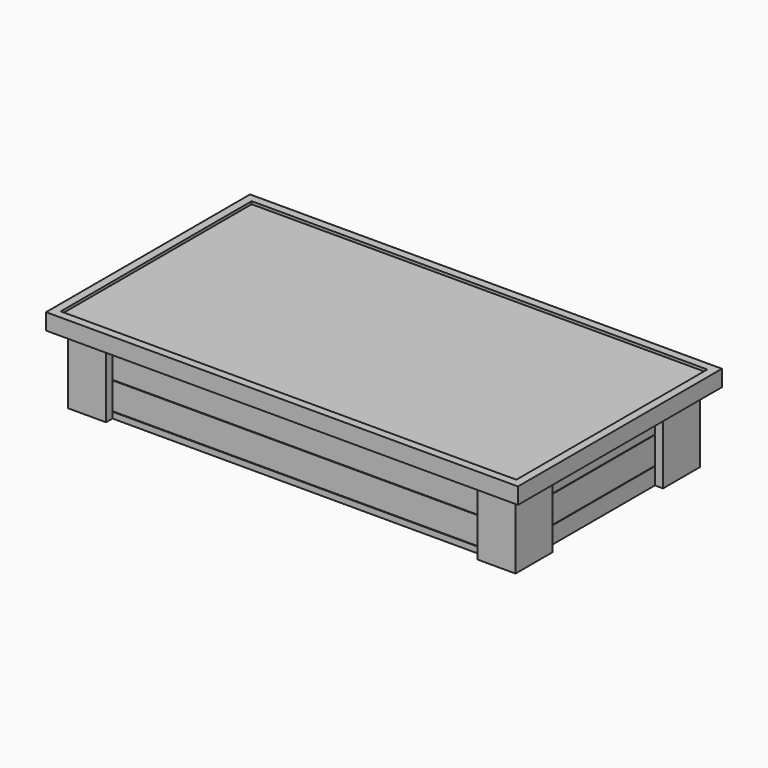
from build123d import *

# Parameters (mm, degrees)
F0_W      = 1066.8
F0_H      = 558.8
F1_DEPTH  = 6.35
F3_W      = 1104.9
F3_H      = 596.9
F3_W_2    = 1066.8
F3_H_2    = 558.8
F4_DEPTH  = 38.1
F5_W      = 1066.8
F5_H      = 558.8
F6_DEPTH  = 19.05
F7_W      = 872.49
F7_H      = 19.05
F8_DEPTH  = 88.9
F9_W      = 38.1
F9_H      = 63.5
F10_DEPTH = 457.2
F11_W     = 19.05
F11_H     = 88.9
F12_DEPTH = 419.1
F14_DEPTH = 192.786
F15_W     = 323.85
F15_H     = 1.143
F15_W_2   = 329.2250932205
F16_DEPTH = 1219.2
F17_W     = 869.95
F17_H     = 1.143
F18_DEPTH = 25.4
F20_W     = 872.49
F20_H     = 19.05
F21_DEPTH = 128.143
F22_W     = 869.95
F22_H     = 1.143
F23_DEPTH = 25.4
F24_W     = 38.1
F24_H     = 88.9
F25_DEPTH = 226.314
F26_W     = 558.8
F26_H     = 381
F27_DEPTH = 1397


# Not quite as in the source:
# - a feature of the source that left no trace in its solid (it failed there, or was rolled back) is left out


with BuildPart() as f1:
    # F0 (on Top) → F1 (new body)
    with BuildSketch(Plane.XY):
        with Locations((32.4463618145, 18.8094943296)):
            Rectangle(F0_W, F0_H)
    extrude(amount=F1_DEPTH)


with BuildPart() as f4:
    # F3 (on offset) → F4 (new body)
    with BuildSketch(Plane.XY.offset(12.7)):
        with Locations((32.4463618145, 18.8094943296)):
            Rectangle(F3_W, F3_H)
        with Locations((32.4463618145, 18.8094943296)):
            Rectangle(F3_W_2, F3_H_2, mode=Mode.SUBTRACT)
    extrude(amount=-F4_DEPTH)


with BuildPart() as f6:
    # F5 (on face) → F6 (new body)
    with BuildSketch(Plane(origin=(0, 0, 0), x_dir=(1, 0, 0), z_dir=(0, 0, -1))):
        with Locations((32.4463618145, -18.8094943296)):
            Rectangle(F5_W, F5_H)
        Polygon((-462.8536381855, -233.1854943296), (-462.8536381855, 195.5665056704), (-9.4854419759, -18.8094943296), align=None, mode=Mode.SUBTRACT)
        Polygon((32.4463618145, -38.6370262221), (500.8223618145, -260.1094943296), (-435.9296381855, -260.1094943296), align=None, mode=Mode.SUBTRACT)
        Polygon((-435.9296381855, 222.4905056704), (500.8223618145, 222.4905056704), (32.4463618145, 1.0180375628), align=None, mode=Mode.SUBTRACT)
        Polygon((74.378165605, -18.8094943296), (527.7463618145, 195.5665056704), (527.7463618145, -233.1854943296), align=None, mode=Mode.SUBTRACT)
    extrude(amount=F6_DEPTH)

    # F7 (on face) → F8 (join)
    with BuildSketch(Plane(origin=(0, 0, -19.05), x_dir=(1, 0, 0), z_dir=(0, 0, -1))):
        with Locations((32.4463618145, 222.4905056704)):
            Rectangle(F7_W, F7_H)
    extrude(amount=F8_DEPTH)

    # F9 (on face) → F10 (join)
    with BuildSketch(Plane(origin=(0, -212.9655056704, 0), x_dir=(-1, 0, 0), z_dir=(0, 1, 0))):
        with Locations((384.7486381855, -50.8)):
            Rectangle(F9_W, F9_H)
        with Locations((-449.6413618145, -50.8)):
            Rectangle(F9_W, F9_H)
    extrude(amount=F10_DEPTH)

    # F11 (on face) → F12 (join)
    with BuildSketch(Plane(origin=(0, 0, -19.05), x_dir=(1, 0, 0), z_dir=(0, 0, -1))):
        Polygon((-402.5286381855, 251.0655056704), (-491.4286381855, 251.0655056704), (-491.4286381855, 232.0155056704), (-472.3786381855, 232.0155056704), (-402.5286381855, 232.0155056704), align=None)
        with Locations((-481.9036381855, 187.5655056704)):
            Rectangle(F11_W, F11_H)
        Polygon((-491.4286381855, -269.6344943296), (-491.4286381855, -288.6844943296), (-402.5286381855, -288.6844943296), (-402.5286381855, -269.6344943296), (-472.3786381855, -269.6344943296), align=None)
        with Locations((-481.9036381855, -225.1844943296)):
            Rectangle(F11_W, F11_H)
        Polygon((467.4213618145, -288.6844943296), (556.3213618145, -288.6844943296), (556.3213618145, -269.6344943296), (537.2713618145, -269.6344943296), (467.4213618145, -269.6344943296), align=None)
        with Locations((546.7963618145, -225.1844943296)):
            Rectangle(F11_W, F11_H)
        with Locations((546.7963618145, 187.5655056704)):
            Rectangle(F11_W, F11_H)
        Polygon((537.2713618145, 232.0155056704), (556.3213618145, 232.0155056704), (556.3213618145, 251.0655056704), (467.4213618145, 251.0655056704), (467.4213618145, 232.0155056704), align=None)
    extrude(amount=F12_DEPTH)

    # F13 (on face) → F14 (join)
    with BuildSketch(Plane(origin=(0, 0, -19.05), x_dir=(1, 0, 0), z_dir=(0, 0, -1))):
        Polygon((-453.3286381855, 232.0155056704), (-472.3786381855, 232.0155056704), (-472.3786381855, -269.6344943296), (537.2713618145, -269.6344943296), (537.2713618145, 232.0155056704), (518.2213618145, 232.0155056704), (518.2213618145, 212.9655056704), (518.2213618145, -250.5844943296), (-453.3286381855, -250.5844943296), (-453.3286381855, 212.9655056704), align=None)
    extrude(amount=F14_DEPTH)

    # F15 (on face) → F16 (cut)
    with BuildSketch(Plane.YZ.offset(537.2713618145)):
        with Locations((18.8094943296, -83.1215)):
            Rectangle(F15_W, F15_H)
        with Locations((21.4970409399, -147.7645)):
            Rectangle(F15_W_2, F15_H)
    extrude(amount=-F16_DEPTH, mode=Mode.SUBTRACT)

    # F17 (on face) → F18 (cut)
    with BuildSketch(Plane(origin=(0, 269.6344943296, 0), x_dir=(-1, 0, 0), z_dir=(0, 1, 0))):
        with Locations((-32.4463618145, -147.7645)):
            Rectangle(F17_W, F17_H)
        with Locations((-32.4463618145, -83.1215)):
            Rectangle(F17_W, F17_H)
    extrude(amount=-F18_DEPTH, mode=Mode.SUBTRACT)

    # F20 (on offset) → F21 (join)
    with BuildSketch(Plane(origin=(0, 0, -109.093), x_dir=(1, 0, 0), z_dir=(0, 0, -1))):
        with Locations((32.4463618145, 222.4905056704)):
            Rectangle(F20_W, F20_H)
    extrude(amount=F21_DEPTH)

    # F22 (on face) → F23 (cut)
    with BuildSketch(Plane.XZ.offset(232.0155056704)):
        with Locations((32.4463618145, -173.1645)):
            Rectangle(F22_W, F22_H)
    extrude(amount=-F23_DEPTH, mode=Mode.SUBTRACT)

    # F24 (on face) → F25 (join, through all)
    with BuildSketch(Plane(origin=(0, 0, -211.836), x_dir=(1, 0, 0), z_dir=(0, 0, -1))):
        with Locations((-453.3286381855, -225.1844943296)):
            Rectangle(F24_W, F24_H)
        with Locations((-453.3286381855, 187.5655056704)):
            Rectangle(F24_W, F24_H)
        with Locations((518.2213618145, -225.1844943296)):
            Rectangle(F24_W, F24_H)
        with Locations((518.2213618145, 187.5655056704)):
            Rectangle(F24_W, F24_H)
    extrude(amount=F25_DEPTH)

    # F26 (on face) → F27 (cut)
    with BuildSketch(Plane(origin=(-491.4286381855, 0, 0), x_dir=(0, -1, 0), z_dir=(-1, 0, 0))):
        with Locations((-15.6344943296, -378.333)):
            Rectangle(F26_W, F26_H)
    extrude(amount=-F27_DEPTH, mode=Mode.SUBTRACT)


solid = Compound([f1.part, f4.part, f6.part])
